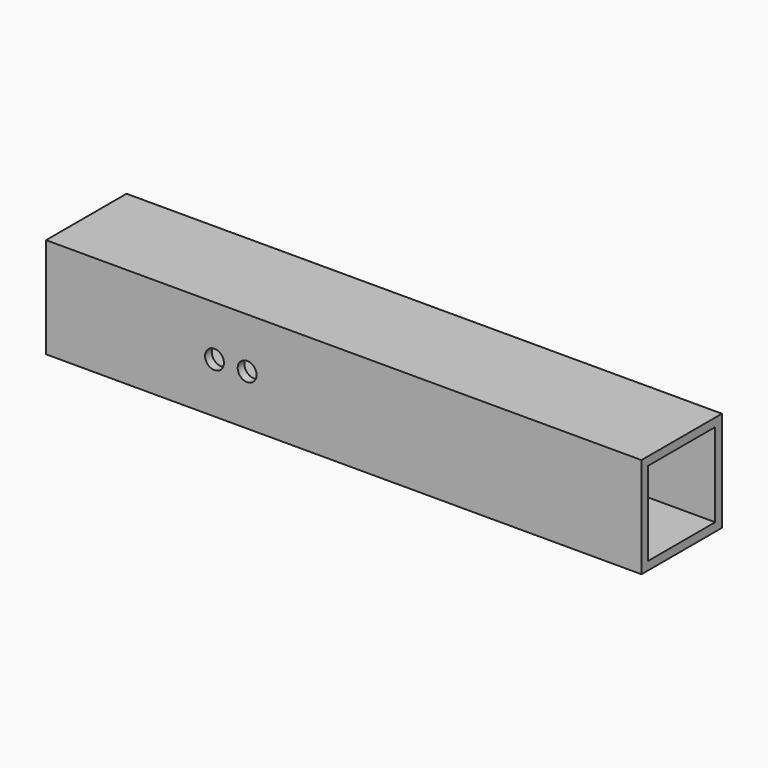
from build123d import *

# Parameters (mm, degrees)
F1_W     = 76.2
F1_H     = 76.2
F1_W_2   = 63.5
F1_H_2   = 63.5
F2_DEPTH = 451.32752
F3_R     = 7.14375
F4_DEPTH = 76.201


# Not quite as in the source:
# - a variable given as a bare number and used for a length is read in inches; the dataset says mm whatever the document's units were


with BuildPart() as f2:
    # F1 (on Right) → F2 (new body)
    with BuildSketch(Plane.YZ):
        Rectangle(F1_W, F1_H)
        Rectangle(F1_W_2, F1_H_2, mode=Mode.SUBTRACT)
    extrude(amount=F2_DEPTH)

    # F3 (on face) → F4 (cut, through all)
    with BuildSketch(Plane.XZ.offset(38.1)):
        with Locations((152.4, 0)):
            Circle(F3_R)
        with Locations((127.6604, 0)):
            Circle(F3_R)
    extrude(amount=-F4_DEPTH, mode=Mode.SUBTRACT)


solid = f2.part
